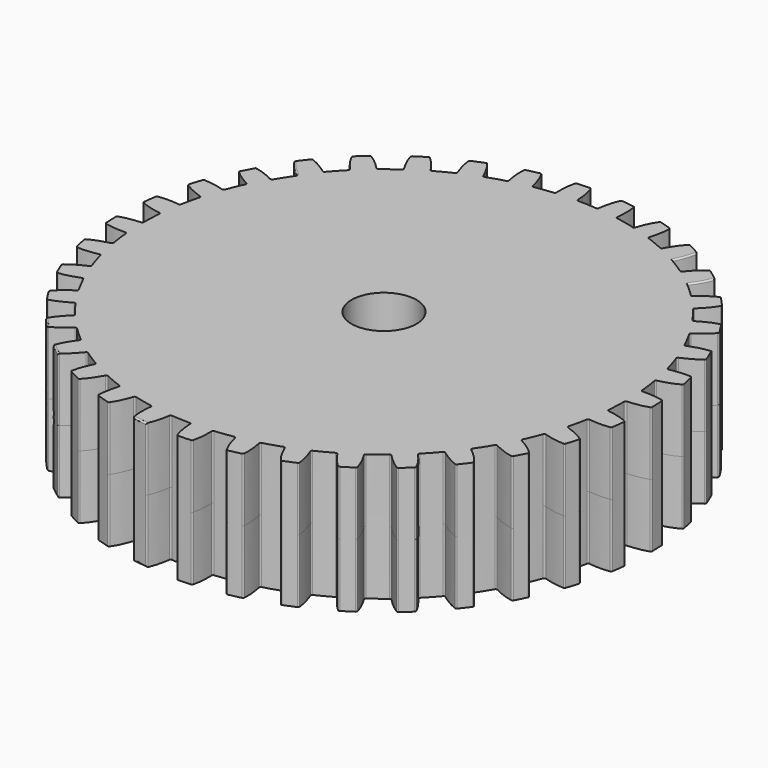
from build123d import *

# Parameters (mm, degrees)
F0_R     = 6.4021431983
F1_DEPTH = 12.5
F2_R     = 0.3


# Not quite as in the source:
# - the dataset's text gives a spline's control points without its knots; the knots are read off the source's solid


with BuildPart() as f1:
    # F0 (on Top) → F1 (new body, symmetric)
    with BuildSketch(Plane.XY):
        with BuildLine():
            ThreePointArc((47.3191638468, -4.1408613644), (47.4547694269, -2.0724040722), (47.5, 0))
            ThreePointArc((47.5, 0), (47.4999999975, 0.0004836327), (47.4999999902, 0.0009672655))
            ThreePointArc((47.4999999902, 0.0009672655), (47.4547905251, 2.0719208999), (47.3193324523, 4.1389341949))
            ThreePointArc((47.3193324523, 4.1389341949), (47.0936309153, 6.1999941305), (46.7782002945, 8.249241008))
            ThreePointArc((46.7782002945, 8.249241008), (46.3740603382, 10.2808816621), (45.8817270859, 12.2929703331))
            ThreePointArc((45.8817270859, 12.2929703331), (45.3015551605, 14.2835254765), (44.6350686538, 16.2468657368))
            ThreePointArc((44.6350686538, 16.2468657368), (43.8842777943, 18.1774630373), (43.0500286594, 20.0734907883))
            ThreePointArc((43.0500286594, 20.0734907883), (42.133014576, 21.9330591287), (41.1357230385, 23.7508376716))
            ThreePointArc((41.1357230385, 23.7508376716), (40.0610936761, 25.5217313965), (38.9102768963, 27.2440883835))
            ThreePointArc((38.9102768963, 27.2440883835), (37.6842836638, 28.9161678779), (36.3864892943, 30.5331524221))
            ThreePointArc((36.3864892943, 30.5331524221), (35.0206734985, 32.0905348617), (33.5882560594, 33.5868881394))
            ThreePointArc((33.5882560594, 33.5868881394), (32.0905348617, 35.0206734985), (30.5316704854, 36.3877327869))
            ThreePointArc((30.5316704854, 36.3877327869), (28.9161678779, 37.6842836638), (27.2456730585, 38.909167295))
            ThreePointArc((27.2456730585, 38.909167295), (25.5217313965, 40.0610936761), (23.7491623186, 41.136690304))
            ThreePointArc((23.7491623186, 41.136690304), (21.9330591287, 42.133014576), (20.0752440688, 43.0492110913))
            ThreePointArc((20.0752440688, 43.0492110913), (18.1774630373, 43.8842777943), (16.2450478724, 44.6357303024))
            ThreePointArc((16.2450478724, 44.6357303024), (14.2835254765, 45.3015551605), (12.2948389465, 45.8812263925))
            ThreePointArc((12.2948389465, 45.8812263925), (10.2808816621, 46.3740603382), (8.2473358669, 46.7785362223))
            ThreePointArc((8.2473358669, 46.7785362223), (6.1999941305, 47.0936309153), (4.1408613644, 47.3191638468))
            ThreePointArc((4.1408613644, 47.3191638468), (2.211991256, 47.4484677801), (0.2794571986, 47.4991779263))
            ThreePointArc((0.2794571986, 47.4991779263), (0.1392455732, 47.4997959014), (-0.0009672655, 47.4999999902))
            ThreePointArc((-0.0009672655, 47.4999999902), (-0.1402128345, 47.499793056), (-0.2794571986, 47.4991779263))
            ThreePointArc((-0.2794571986, 47.4991779263), (-2.2110250395, 47.4485128142), (-4.1389341949, 47.3193324523))
            ThreePointArc((-4.1389341949, 47.3193324523), (-6.1999941305, 47.0936309153), (-8.249241008, 46.7782002945))
            ThreePointArc((-8.249241008, 46.7782002945), (-10.2808816621, 46.3740603382), (-12.2929703331, 45.8817270859))
            ThreePointArc((-12.2929703331, 45.8817270859), (-14.2835254765, 45.3015551605), (-16.2468657368, 44.6350686538))
            ThreePointArc((-16.2468657368, 44.6350686538), (-18.1774630373, 43.8842777943), (-20.0734907883, 43.0500286594))
            ThreePointArc((-20.0734907883, 43.0500286594), (-21.9330591287, 42.133014576), (-23.7508376716, 41.1357230385))
            ThreePointArc((-23.7508376716, 41.1357230385), (-25.5217313965, 40.0610936761), (-27.2440883835, 38.9102768963))
            ThreePointArc((-27.2440883835, 38.9102768963), (-28.9161678779, 37.6842836638), (-30.5331524221, 36.3864892943))
            ThreePointArc((-30.5331524221, 36.3864892943), (-32.0905348617, 35.0206734985), (-33.5868881394, 33.5882560594))
            ThreePointArc((-33.5868881394, 33.5882560594), (-35.0206734985, 32.0905348617), (-36.3877327869, 30.5316704854))
            ThreePointArc((-36.3877327869, 30.5316704854), (-37.6842836638, 28.9161678779), (-38.909167295, 27.2456730585))
            ThreePointArc((-38.909167295, 27.2456730585), (-40.0610936761, 25.5217313965), (-41.136690304, 23.7491623186))
            ThreePointArc((-41.136690304, 23.7491623186), (-42.133014576, 21.9330591287), (-43.0492110913, 20.0752440688))
            ThreePointArc((-43.0492110913, 20.0752440688), (-43.8842777943, 18.1774630373), (-44.6357303024, 16.2450478724))
            ThreePointArc((-44.6357303024, 16.2450478724), (-45.3015551605, 14.2835254765), (-45.8812263925, 12.2948389465))
            ThreePointArc((-45.8812263925, 12.2948389465), (-46.3740603382, 10.2808816621), (-46.7785362223, 8.2473358669))
            ThreePointArc((-46.7785362223, 8.2473358669), (-47.0936309153, 6.1999941305), (-47.3191638468, 4.1408613644))
            ThreePointArc((-47.3191638468, 4.1408613644), (-47.4547905251, 2.0719208999), (-47.4999999902, -0.0009672655))
            ThreePointArc((-47.4999999902, -0.0009672655), (-47.4547905251, -2.0719208999), (-47.3193324523, -4.1389341949))
            ThreePointArc((-47.3193324523, -4.1389341949), (-47.0936309153, -6.1999941305), (-46.7782002945, -8.249241008))
            ThreePointArc((-46.7782002945, -8.249241008), (-46.3740603382, -10.2808816621), (-45.8817270859, -12.2929703331))
            ThreePointArc((-45.8817270859, -12.2929703331), (-45.3015551605, -14.2835254765), (-44.6350686538, -16.2468657368))
            ThreePointArc((-44.6350686538, -16.2468657368), (-43.8842777943, -18.1774630373), (-43.0500286594, -20.0734907883))
            ThreePointArc((-43.0500286594, -20.0734907883), (-42.133014576, -21.9330591287), (-41.1357230385, -23.7508376716))
            ThreePointArc((-41.1357230385, -23.7508376716), (-40.0610936761, -25.5217313965), (-38.9102768963, -27.2440883835))
            ThreePointArc((-38.9102768963, -27.2440883835), (-37.6842836638, -28.9161678779), (-36.3864892943, -30.5331524221))
            ThreePointArc((-36.3864892943, -30.5331524221), (-35.0206734985, -32.0905348617), (-33.5882560594, -33.5868881394))
            ThreePointArc((-33.5882560594, -33.5868881394), (-32.0905348617, -35.0206734985), (-30.5316704854, -36.3877327869))
            ThreePointArc((-30.5316704854, -36.3877327869), (-28.9161678779, -37.6842836638), (-27.2456730585, -38.909167295))
            ThreePointArc((-27.2456730585, -38.909167295), (-25.5217313965, -40.0610936761), (-23.7491623186, -41.136690304))
            ThreePointArc((-23.7491623186, -41.136690304), (-21.9330591287, -42.133014576), (-20.0752440688, -43.0492110913))
            ThreePointArc((-20.0752440688, -43.0492110913), (-18.1774630373, -43.8842777943), (-16.2450478724, -44.6357303024))
            ThreePointArc((-16.2450478724, -44.6357303024), (-14.2835254765, -45.3015551605), (-12.2948389465, -45.8812263925))
            ThreePointArc((-12.2948389465, -45.8812263925), (-10.2808816621, -46.3740603382), (-8.2473358669, -46.7785362223))
            ThreePointArc((-8.2473358669, -46.7785362223), (-6.1999941305, -47.0936309153), (-4.1408613644, -47.3191638468))
            ThreePointArc((-4.1408613644, -47.3191638468), (-2.0719208999, -47.4547905251), (0.0009672655, -47.4999999902))
            ThreePointArc((0.0009672655, -47.4999999902), (2.0719208999, -47.4547905251), (4.1389341949, -47.3193324523))
            ThreePointArc((4.1389341949, -47.3193324523), (6.1999941305, -47.0936309153), (8.249241008, -46.7782002945))
            ThreePointArc((8.249241008, -46.7782002945), (10.2808816621, -46.3740603382), (12.2929703331, -45.8817270859))
            ThreePointArc((12.2929703331, -45.8817270859), (14.2835254765, -45.3015551605), (16.2468657368, -44.6350686538))
            ThreePointArc((16.2468657368, -44.6350686538), (18.1774630373, -43.8842777943), (20.0734907883, -43.0500286594))
            ThreePointArc((20.0734907883, -43.0500286594), (21.9330591287, -42.133014576), (23.7508376716, -41.1357230385))
            ThreePointArc((23.7508376716, -41.1357230385), (25.5217313965, -40.0610936761), (27.2440883835, -38.9102768963))
            ThreePointArc((27.2440883835, -38.9102768963), (28.9161678779, -37.6842836638), (30.5331524221, -36.3864892943))
            ThreePointArc((30.5331524221, -36.3864892943), (32.0905348617, -35.0206734985), (33.5868881394, -33.5882560594))
            ThreePointArc((33.5868881394, -33.5882560594), (35.0206734985, -32.0905348617), (36.3877327869, -30.5316704854))
            ThreePointArc((36.3877327869, -30.5316704854), (37.6842836638, -28.9161678779), (38.909167295, -27.2456730585))
            ThreePointArc((38.909167295, -27.2456730585), (40.0610936761, -25.5217313965), (41.136690304, -23.7491623186))
            ThreePointArc((41.136690304, -23.7491623186), (42.133014576, -21.9330591287), (43.0492110913, -20.0752440688))
            ThreePointArc((43.0492110913, -20.0752440688), (43.8842777943, -18.1774630373), (44.6357303024, -16.2450478724))
            ThreePointArc((44.6357303024, -16.2450478724), (45.3015551605, -14.2835254765), (45.8812263925, -12.2948389465))
            ThreePointArc((45.8812263925, -12.2948389465), (46.3740603382, -10.2808816621), (46.7785362223, -8.2473358669))
            ThreePointArc((46.7785362223, -8.2473358669), (47.0936309153, -6.1999941305), (47.3191638468, -4.1408613644))
        make_face()
        Circle(F0_R, mode=Mode.SUBTRACT)
        with BuildLine():
            ThreePointArc((-43.0492110913, 20.0752440688), (-42.133014576, 21.9330591287), (-41.136690304, 23.7491623186))
            add(Edge.make_bspline(
                [(-45.4369608695, 25.2879929401), (-44.8516797618, 25.1784985185), (-43.3336628589, 24.8141226526), (-41.9586973612, 24.1177232288), (-41.136690304, 23.7491623186)],
                knots=[0.0012573797, 0.0012573797, 0.0012573797, 0.0012573797, 0.4755379839, 1, 1, 1, 1], degree=3))
            ThreePointArc((-45.4369608695, 25.2879929401), (-46.1245633253, 24.0109278882), (-46.7762812071, 22.7151825095))
            add(Edge.make_bspline(
                [(-46.7762812071, 22.7151825095), (-46.3508851757, 22.2985517138), (-45.1817072148, 21.2640624752), (-43.8226023929, 20.5371949767), (-43.0492110913, 20.0752440688)],
                knots=[0.0012573797, 0.0012573797, 0.0012573797, 0.0012573797, 0.4755379839, 1, 1, 1, 1], degree=3))
        make_face()
        with BuildLine():
            ThreePointArc((-45.8812263925, 12.2948389465), (-45.3015551605, 14.2835254765), (-44.6357303024, 16.2450478724))
            add(Edge.make_bspline(
                [(-49.1378852285, 17.0137660519), (-48.5424823492, 17.0075680943), (-46.9842543289, 16.9123287854), (-45.5092491558, 16.4652694867), (-44.6357303024, 16.2450478724)],
                knots=[0.0012573797, 0.0012573797, 0.0012573797, 0.0012573797, 0.4755379839, 1, 1, 1, 1], degree=3))
            ThreePointArc((-49.1378852285, 17.0137660519), (-49.5932814389, 15.6367015742), (-50.0100944379, 14.2474718568))
            add(Edge.make_bspline(
                [(-50.0100944379, 14.2474718568), (-49.5188139498, 13.9110398647), (-48.187761258, 13.0952924644), (-46.7230850757, 12.615473792), (-45.8812263925, 12.2948389465)],
                knots=[0.0012573797, 0.0012573797, 0.0012573797, 0.0012573797, 0.4755379839, 1, 1, 1, 1], degree=3))
        make_face()
        with BuildLine():
            ThreePointArc((-47.3191638468, 4.1408613644), (-47.0936309153, 6.1999941305), (-46.7785362223, 8.2473358669))
            add(Edge.make_bspline(
                [(-51.3457798098, 8.2225844915), (-50.7583461741, 8.3198713198), (-49.2072530063, 8.4966623661), (-47.6770254435, 8.312526863), (-46.7785362223, 8.2473358669)],
                knots=[0.0012573797, 0.0012573797, 0.0012573797, 0.0012573797, 0.4755379839, 1, 1, 1, 1], degree=3))
            ThreePointArc((-51.3457798098, 8.2225844915), (-51.5551327914, 6.7873619954), (-51.7243762556, 5.3468589813))
            add(Edge.make_bspline(
                [(-51.7243762556, 5.3468589813), (-51.1821386196, 5.1008481086), (-49.7296545597, 4.5286286186), (-48.2039104616, 4.3104378199), (-47.3191638468, 4.1408613644)],
                knots=[0.0012573797, 0.0012573797, 0.0012573797, 0.0012573797, 0.4755379839, 1, 1, 1, 1], degree=3))
        make_face()
        with BuildLine():
            add(Edge.make_bspline(
                [(-51.8670390746, -3.7162154987), (-51.290319907, -3.8643303361), (-49.7605374719, -4.1756353162), (-48.2200844205, -4.1255686242), (-47.3193324523, -4.1389341949)],
                knots=[0.0012573797, 0.0012573797, 0.0012573797, 0.0012573797, 0.4755379839, 1, 1, 1, 1], degree=3))
            ThreePointArc((-47.3193324523, -4.1389341949), (-47.4547905251, -2.0719208999), (-47.4999999902, -0.0009672655))
            add(Edge.make_bspline(
                [(-51.9935588538, -0.8184361379), (-51.4319433354, -0.6206205347), (-49.9351142012, -0.1771708397), (-48.3961594389, -0.092787683), (-47.4999999902, -0.0009672655)],
                knots=[0.0012573797, 0.0012573797, 0.0012573797, 0.0012573797, 0.4755379839, 1, 1, 1, 1], degree=3))
            ThreePointArc((-51.9935588538, -0.8184361379), (-51.9505075223, -2.268208143), (-51.8670390746, -3.7162154987))
        make_face()
        with BuildLine():
            add(Edge.make_bspline(
                [(-50.4337481573, -12.6663746513), (-49.8400707781, -12.712093059), (-48.2794716332, -12.7530246849), (-46.7711155148, -12.4362217532), (-45.8817270859, -12.2929703331)],
                knots=[0.0012573797, 0.0012573797, 0.0012573797, 0.0012573797, 0.4755379839, 1, 1, 1, 1], degree=3))
            ThreePointArc((-45.8817270859, -12.2929703331), (-46.3740603382, -10.2808816621), (-46.7782002945, -8.249241008))
            add(Edge.make_bspline(
                [(-51.0615399221, -9.8345889993), (-50.5428069243, -9.5422551483), (-49.1457222194, -8.8456207992), (-47.6448006194, -8.4952829223), (-46.7782002945, -8.249241008)],
                knots=[0.0012573797, 0.0012573797, 0.0012573797, 0.0012573797, 0.4755379839, 1, 1, 1, 1], degree=3))
            ThreePointArc((-51.0615399221, -9.8345889993), (-50.7673923702, -11.2548599248), (-50.4337481573, -12.6663746513))
        make_face()
        with BuildLine():
            add(Edge.make_bspline(
                [(-47.4680533229, -21.2316724196), (-46.8754563189, -21.173605267), (-45.3314584794, -20.9429198518), (-43.9010299315, -20.3690065773), (-43.0500286594, -20.0734907883)],
                knots=[0.0012573797, 0.0012573797, 0.0012573797, 0.0012573797, 0.4755379839, 1, 1, 1, 1], degree=3))
            ThreePointArc((-43.0500286594, -20.0734907883), (-43.8842777943, -18.1774630373), (-44.6350686538, -16.2468657368))
            add(Edge.make_bspline(
                [(-48.5780419382, -18.5519228506), (-48.1179529007, -18.1739531679), (-46.8630623369, -17.2453010468), (-45.4457786425, -16.6396532887), (-44.6350686538, -16.2468657368)],
                knots=[0.0012573797, 0.0012573797, 0.0012573797, 0.0012573797, 0.4755379839, 1, 1, 1, 1], degree=3))
            ThreePointArc((-48.5780419382, -18.5519228506), (-48.0417356906, -19.899538483), (-47.4680533229, -21.2316724196))
        make_face()
        with BuildLine():
            add(Edge.make_bspline(
                [(-43.0600657083, -29.1518565651), (-42.4865548396, -28.9917681932), (-41.0060718986, -28.4964749967), (-39.6970337687, -27.6828894438), (-38.9102768963, -27.2440883835)],
                knots=[0.0012573797, 0.0012573797, 0.0012573797, 0.0012573797, 0.4755379839, 1, 1, 1, 1], degree=3))
            ThreePointArc((-38.9102768963, -27.2440883835), (-40.0610936761, -25.5217313965), (-41.1357230385, -23.7508376716))
            add(Edge.make_bspline(
                [(-44.6185247317, -26.7055659137), (-44.2310592271, -26.2534448169), (-43.1564920192, -25.1209915486), (-41.8659096782, -24.2784362101), (-41.1357230385, -23.7508376716)],
                knots=[0.0012573797, 0.0012573797, 0.0012573797, 0.0012573797, 0.4755379839, 1, 1, 1, 1], degree=3))
            ThreePointArc((-44.6185247317, -26.7055659137), (-43.8563551823, -27.939579634), (-43.0600657083, -29.1518565651))
        make_face()
        with BuildLine():
            add(Edge.make_bspline(
                [(-37.3437197866, -36.1862763005), (-36.8067208907, -35.9290309134), (-35.4347365732, -35.1841791688), (-34.2868633225, -34.1556417228), (-33.5882560594, -33.5868881394)],
                knots=[0.0012573797, 0.0012573797, 0.0012573797, 0.0012573797, 0.4755379839, 1, 1, 1, 1], degree=3))
            ThreePointArc((-33.5882560594, -33.5868881394), (-35.0206734985, -32.0905348617), (-36.3864892943, -30.5331524221))
            add(Edge.make_bspline(
                [(-39.3032962292, -34.0477738702), (-39.0002272009, -33.53523883), (-38.1386335297, -32.233393434), (-37.0139662335, -31.1795311327), (-36.3864892943, -30.5331524221)],
                knots=[0.0012573797, 0.0012573797, 0.0012573797, 0.0012573797, 0.4755379839, 1, 1, 1, 1], degree=3))
            ThreePointArc((-39.3032962292, -34.0477738702), (-38.3384215141, -35.130690796), (-37.3437197866, -36.1862763005))
        make_face()
        with BuildLine():
            add(Edge.make_bspline(
                [(-30.4927038361, -42.1211943416), (-30.0085333527, -41.7746082103), (-28.7867347078, -40.8028298608), (-27.8349038843, -39.5905921116), (-27.2456730585, -38.909167295)],
                knots=[0.0012573797, 0.0012573797, 0.0012573797, 0.0012573797, 0.4755379839, 1, 1, 1, 1], degree=3))
            ThreePointArc((-27.2456730585, -38.909167295), (-28.9161678779, -37.6842836638), (-30.5316704854, -36.3877327869))
            add(Edge.make_bspline(
                [(-32.7938569593, -40.3554574467), (-32.5843930062, -39.798081581), (-31.9619519595, -38.3663999709), (-31.0373721548, -37.1332517795), (-30.5316704854, -36.3877327869)],
                knots=[0.0012573797, 0.0012573797, 0.0012573797, 0.0012573797, 0.4755379839, 1, 1, 1, 1], degree=3))
            ThreePointArc((-32.7938569593, -40.3554574467), (-31.6555943085, -41.2543736951), (-30.4927038361, -42.1211943416))
        make_face()
        with BuildLine():
            add(Edge.make_bspline(
                [(-22.7151825095, -46.7762812071), (-22.2985517138, -46.3508851757), (-21.2640624752, -45.1817072148), (-20.5371949767, -43.8226023929), (-20.0752440688, -43.0492110913)],
                knots=[0.0012573797, 0.0012573797, 0.0012573797, 0.0012573797, 0.4755379839, 1, 1, 1, 1], degree=3))
            ThreePointArc((-20.0752440688, -43.0492110913), (-21.9330591287, -42.133014576), (-23.7491623186, -41.136690304))
            add(Edge.make_bspline(
                [(-25.2879929401, -45.4369608695), (-25.1784985185, -44.8516797618), (-24.8141226526, -43.3336628589), (-24.1177232288, -41.9586973612), (-23.7491623186, -41.136690304)],
                knots=[0.0012573797, 0.0012573797, 0.0012573797, 0.0012573797, 0.4755379839, 1, 1, 1, 1], degree=3))
            ThreePointArc((-25.2879929401, -45.4369608695), (-24.0109278882, -46.1245633253), (-22.7151825095, -46.7762812071))
        make_face()
        with BuildLine():
            add(Edge.make_bspline(
                [(-14.2474718568, -50.0100944379), (-13.9110398647, -49.5188139498), (-13.0952924644, -48.187761258), (-12.615473792, -46.7230850757), (-12.2948389465, -45.8812263925)],
                knots=[0.0012573797, 0.0012573797, 0.0012573797, 0.0012573797, 0.4755379839, 1, 1, 1, 1], degree=3))
            ThreePointArc((-12.2948389465, -45.8812263925), (-14.2835254765, -45.3015551605), (-16.2450478724, -44.6357303024))
            add(Edge.make_bspline(
                [(-17.0137660519, -49.1378852285), (-17.0075680943, -48.5424823492), (-16.9123287854, -46.9842543289), (-16.4652694867, -45.5092491558), (-16.2450478724, -44.6357303024)],
                knots=[0.0012573797, 0.0012573797, 0.0012573797, 0.0012573797, 0.4755379839, 1, 1, 1, 1], degree=3))
            ThreePointArc((-17.0137660519, -49.1378852285), (-15.6367015742, -49.5932814389), (-14.2474718568, -50.0100944379))
        make_face()
        with BuildLine():
            add(Edge.make_bspline(
                [(-5.3468589813, -51.7243762556), (-5.1008481086, -51.1821386196), (-4.5286286186, -49.7296545597), (-4.3104378199, -48.2039104616), (-4.1408613644, -47.3191638468)],
                knots=[0.0012573797, 0.0012573797, 0.0012573797, 0.0012573797, 0.4755379839, 1, 1, 1, 1], degree=3))
            ThreePointArc((-4.1408613644, -47.3191638468), (-6.1999941305, -47.0936309153), (-8.2473358669, -46.7785362223))
            add(Edge.make_bspline(
                [(-8.2225844915, -51.3457798098), (-8.3198713198, -50.7583461741), (-8.4966623661, -49.2072530063), (-8.312526863, -47.6770254435), (-8.2473358669, -46.7785362223)],
                knots=[0.0012573797, 0.0012573797, 0.0012573797, 0.0012573797, 0.4755379839, 1, 1, 1, 1], degree=3))
            ThreePointArc((-8.2225844915, -51.3457798098), (-6.7873619954, -51.5551327914), (-5.3468589813, -51.7243762556))
        make_face()
        with BuildLine():
            add(Edge.make_bspline(
                [(3.7162154987, -51.8670390746), (3.8643303361, -51.290319907), (4.1756353162, -49.7605374719), (4.1255686242, -48.2200844205), (4.1389341949, -47.3193324523)],
                knots=[0.0012573797, 0.0012573797, 0.0012573797, 0.0012573797, 0.4755379839, 1, 1, 1, 1], degree=3))
            ThreePointArc((4.1389341949, -47.3193324523), (2.0719208999, -47.4547905251), (0.0009672655, -47.4999999902))
            add(Edge.make_bspline(
                [(0.8184361379, -51.9935588538), (0.6206205347, -51.4319433354), (0.1771708397, -49.9351142012), (0.092787683, -48.3961594389), (0.0009672655, -47.4999999902)],
                knots=[0.0012573797, 0.0012573797, 0.0012573797, 0.0012573797, 0.4755379839, 1, 1, 1, 1], degree=3))
            ThreePointArc((0.8184361379, -51.9935588538), (2.268208143, -51.9505075223), (3.7162154987, -51.8670390746))
        make_face()
        with BuildLine():
            add(Edge.make_bspline(
                [(12.6663746513, -50.4337481573), (12.712093059, -49.8400707781), (12.7530246849, -48.2794716332), (12.4362217532, -46.7711155148), (12.2929703331, -45.8817270859)],
                knots=[0.0012573797, 0.0012573797, 0.0012573797, 0.0012573797, 0.4755379839, 1, 1, 1, 1], degree=3))
            ThreePointArc((12.2929703331, -45.8817270859), (10.2808816621, -46.3740603382), (8.249241008, -46.7782002945))
            add(Edge.make_bspline(
                [(9.8345889993, -51.0615399221), (9.5422551483, -50.5428069243), (8.8456207992, -49.1457222194), (8.4952829223, -47.6448006194), (8.249241008, -46.7782002945)],
                knots=[0.0012573797, 0.0012573797, 0.0012573797, 0.0012573797, 0.4755379839, 1, 1, 1, 1], degree=3))
            ThreePointArc((9.8345889993, -51.0615399221), (11.2548599248, -50.7673923702), (12.6663746513, -50.4337481573))
        make_face()
        with BuildLine():
            add(Edge.make_bspline(
                [(21.2316724196, -47.4680533229), (21.173605267, -46.8754563189), (20.9429198518, -45.3314584794), (20.3690065773, -43.9010299315), (20.0734907883, -43.0500286594)],
                knots=[0.0012573797, 0.0012573797, 0.0012573797, 0.0012573797, 0.4755379839, 1, 1, 1, 1], degree=3))
            ThreePointArc((20.0734907883, -43.0500286594), (18.1774630373, -43.8842777943), (16.2468657368, -44.6350686538))
            add(Edge.make_bspline(
                [(18.5519228506, -48.5780419382), (18.1739531679, -48.1179529007), (17.2453010468, -46.8630623369), (16.6396532887, -45.4457786425), (16.2468657368, -44.6350686538)],
                knots=[0.0012573797, 0.0012573797, 0.0012573797, 0.0012573797, 0.4755379839, 1, 1, 1, 1], degree=3))
            ThreePointArc((18.5519228506, -48.5780419382), (19.899538483, -48.0417356906), (21.2316724196, -47.4680533229))
        make_face()
        with BuildLine():
            add(Edge.make_bspline(
                [(29.1518565651, -43.0600657083), (28.9917681932, -42.4865548396), (28.4964749967, -41.0060718986), (27.6828894438, -39.6970337687), (27.2440883835, -38.9102768963)],
                knots=[0.0012573797, 0.0012573797, 0.0012573797, 0.0012573797, 0.4755379839, 1, 1, 1, 1], degree=3))
            ThreePointArc((27.2440883835, -38.9102768963), (25.5217313965, -40.0610936761), (23.7508376716, -41.1357230385))
            add(Edge.make_bspline(
                [(26.7055659137, -44.6185247317), (26.2534448169, -44.2310592271), (25.1209915486, -43.1564920192), (24.2784362101, -41.8659096782), (23.7508376716, -41.1357230385)],
                knots=[0.0012573797, 0.0012573797, 0.0012573797, 0.0012573797, 0.4755379839, 1, 1, 1, 1], degree=3))
            ThreePointArc((26.7055659137, -44.6185247317), (27.939579634, -43.8563551823), (29.1518565651, -43.0600657083))
        make_face()
        with BuildLine():
            add(Edge.make_bspline(
                [(36.1862763005, -37.3437197866), (35.9290309134, -36.8067208907), (35.1841791688, -35.4347365732), (34.1556417228, -34.2868633225), (33.5868881394, -33.5882560594)],
                knots=[0.0012573797, 0.0012573797, 0.0012573797, 0.0012573797, 0.4755379839, 1, 1, 1, 1], degree=3))
            ThreePointArc((33.5868881394, -33.5882560594), (32.0905348617, -35.0206734985), (30.5331524221, -36.3864892943))
            add(Edge.make_bspline(
                [(34.0477738702, -39.3032962292), (33.53523883, -39.0002272009), (32.233393434, -38.1386335297), (31.1795311327, -37.0139662335), (30.5331524221, -36.3864892943)],
                knots=[0.0012573797, 0.0012573797, 0.0012573797, 0.0012573797, 0.4755379839, 1, 1, 1, 1], degree=3))
            ThreePointArc((34.0477738702, -39.3032962292), (35.130690796, -38.3384215141), (36.1862763005, -37.3437197866))
        make_face()
        with BuildLine():
            add(Edge.make_bspline(
                [(42.1211943416, -30.4927038361), (41.7746082103, -30.0085333527), (40.8028298608, -28.7867347078), (39.5905921116, -27.8349038843), (38.909167295, -27.2456730585)],
                knots=[0.0012573797, 0.0012573797, 0.0012573797, 0.0012573797, 0.4755379839, 1, 1, 1, 1], degree=3))
            ThreePointArc((38.909167295, -27.2456730585), (37.6842836638, -28.9161678779), (36.3877327869, -30.5316704854))
            add(Edge.make_bspline(
                [(40.3554574467, -32.7938569593), (39.798081581, -32.5843930062), (38.3663999709, -31.9619519595), (37.1332517795, -31.0373721548), (36.3877327869, -30.5316704854)],
                knots=[0.0012573797, 0.0012573797, 0.0012573797, 0.0012573797, 0.4755379839, 1, 1, 1, 1], degree=3))
            ThreePointArc((40.3554574467, -32.7938569593), (41.2543736951, -31.6555943085), (42.1211943416, -30.4927038361))
        make_face()
        with BuildLine():
            ThreePointArc((-27.2440883835, 38.9102768963), (-25.5217313965, 40.0610936761), (-23.7508376716, 41.1357230385))
            add(Edge.make_bspline(
                [(-26.7055659137, 44.6185247317), (-26.2534448169, 44.2310592271), (-25.1209915486, 43.1564920192), (-24.2784362101, 41.8659096782), (-23.7508376716, 41.1357230385)],
                knots=[0.0012573797, 0.0012573797, 0.0012573797, 0.0012573797, 0.4755379839, 1, 1, 1, 1], degree=3))
            ThreePointArc((-26.7055659137, 44.6185247317), (-27.939579634, 43.8563551823), (-29.1518565651, 43.0600657083))
            add(Edge.make_bspline(
                [(-29.1518565651, 43.0600657083), (-28.9917681932, 42.4865548396), (-28.4964749967, 41.0060718986), (-27.6828894438, 39.6970337687), (-27.2440883835, 38.9102768963)],
                knots=[0.0012573797, 0.0012573797, 0.0012573797, 0.0012573797, 0.4755379839, 1, 1, 1, 1], degree=3))
        make_face()
        with BuildLine():
            add(Edge.make_bspline(
                [(50.0100944379, -14.2474718568), (49.5188139498, -13.9110398647), (48.187761258, -13.0952924644), (46.7230850757, -12.615473792), (45.8812263925, -12.2948389465)],
                knots=[0.0012573797, 0.0012573797, 0.0012573797, 0.0012573797, 0.4755379839, 1, 1, 1, 1], degree=3))
            ThreePointArc((45.8812263925, -12.2948389465), (45.3015551605, -14.2835254765), (44.6357303024, -16.2450478724))
            add(Edge.make_bspline(
                [(49.1378852285, -17.0137660519), (48.5424823492, -17.0075680943), (46.9842543289, -16.9123287854), (45.5092491558, -16.4652694867), (44.6357303024, -16.2450478724)],
                knots=[0.0012573797, 0.0012573797, 0.0012573797, 0.0012573797, 0.4755379839, 1, 1, 1, 1], degree=3))
            ThreePointArc((49.1378852285, -17.0137660519), (49.5932814389, -15.6367015742), (50.0100944379, -14.2474718568))
        make_face()
        with BuildLine():
            ThreePointArc((12.2948389465, 45.8812263925), (14.2835254765, 45.3015551605), (16.2450478724, 44.6357303024))
            add(Edge.make_bspline(
                [(17.0137660519, 49.1378852285), (17.0075680943, 48.5424823492), (16.9123287854, 46.9842543289), (16.4652694867, 45.5092491558), (16.2450478724, 44.6357303024)],
                knots=[0.0012573797, 0.0012573797, 0.0012573797, 0.0012573797, 0.4755379839, 1, 1, 1, 1], degree=3))
            ThreePointArc((17.0137660519, 49.1378852285), (15.6367015742, 49.5932814389), (14.2474718568, 50.0100944379))
            add(Edge.make_bspline(
                [(14.2474718568, 50.0100944379), (13.9110398647, 49.5188139498), (13.0952924644, 48.187761258), (12.615473792, 46.7230850757), (12.2948389465, 45.8812263925)],
                knots=[0.0012573797, 0.0012573797, 0.0012573797, 0.0012573797, 0.4755379839, 1, 1, 1, 1], degree=3))
        make_face()
        with BuildLine():
            ThreePointArc((-4.1389341949, 47.3193324523), (-2.2110250395, 47.4485128142), (-0.2794571986, 47.4991779263))
            add(Edge.make_bspline(
                [(-0.1401693003, 48.9738556219), (-0.1894884148, 48.5017472335), (-0.2266014064, 48.0150459528), (-0.2794571986, 47.4991779263)],
                knots=[0.6980970455, 0.6980970455, 0.6980970455, 0.6980970455, 1, 1, 1, 1], degree=3))
            add(Edge.make_bspline(
                [(-0.8184361379, 51.9935588538), (-0.6206205347, 51.4319433354), (-0.3111403588, 50.387317645), (-0.17654491, 49.3221745068), (-0.1401693003, 48.9738556219)],
                knots=[0.0012573797, 0.0012573797, 0.0012573797, 0.0012573797, 0.4755379839, 0.698272273, 0.698272273, 0.698272273, 0.698272273], degree=3))
            ThreePointArc((-0.8184361379, 51.9935588538), (-2.268208143, 51.9505075223), (-3.7162154987, 51.8670390746))
            add(Edge.make_bspline(
                [(-3.7162154987, 51.8670390746), (-3.8643303361, 51.290319907), (-4.1756353162, 49.7605374719), (-4.1255686242, 48.2200844205), (-4.1389341949, 47.3193324523)],
                knots=[0.0012573797, 0.0012573797, 0.0012573797, 0.0012573797, 0.4755379839, 1, 1, 1, 1], degree=3))
        make_face()
        with BuildLine():
            ThreePointArc((-12.2929703331, 45.8817270859), (-10.2808816621, 46.3740603382), (-8.249241008, 46.7782002945))
            add(Edge.make_bspline(
                [(-9.8345889993, 51.0615399221), (-9.5422551483, 50.5428069243), (-8.8456207992, 49.1457222194), (-8.4952829223, 47.6448006194), (-8.249241008, 46.7782002945)],
                knots=[0.0012573797, 0.0012573797, 0.0012573797, 0.0012573797, 0.4755379839, 1, 1, 1, 1], degree=3))
            ThreePointArc((-9.8345889993, 51.0615399221), (-11.2548599248, 50.7673923702), (-12.6663746513, 50.4337481573))
            add(Edge.make_bspline(
                [(-12.6663746513, 50.4337481573), (-12.712093059, 49.8400707781), (-12.7530246849, 48.2794716332), (-12.4362217532, 46.7711155148), (-12.2929703331, 45.8817270859)],
                knots=[0.0012573797, 0.0012573797, 0.0012573797, 0.0012573797, 0.4755379839, 1, 1, 1, 1], degree=3))
        make_face()
        with BuildLine():
            ThreePointArc((-38.909167295, 27.2456730585), (-37.6842836638, 28.9161678779), (-36.3877327869, 30.5316704854))
            add(Edge.make_bspline(
                [(-40.3554574467, 32.7938569593), (-39.798081581, 32.5843930062), (-38.3663999709, 31.9619519595), (-37.1332517795, 31.0373721548), (-36.3877327869, 30.5316704854)],
                knots=[0.0012573797, 0.0012573797, 0.0012573797, 0.0012573797, 0.4755379839, 1, 1, 1, 1], degree=3))
            ThreePointArc((-40.3554574467, 32.7938569593), (-41.2543736951, 31.6555943085), (-42.1211943416, 30.4927038361))
            add(Edge.make_bspline(
                [(-42.1211943416, 30.4927038361), (-41.7746082103, 30.0085333527), (-40.8028298608, 28.7867347078), (-39.5905921116, 27.8349038843), (-38.909167295, 27.2456730585)],
                knots=[0.0012573797, 0.0012573797, 0.0012573797, 0.0012573797, 0.4755379839, 1, 1, 1, 1], degree=3))
        make_face()
        with BuildLine():
            ThreePointArc((-0.2794571986, 47.4991779263), (-0.1402128345, 47.499793056), (-0.0009672655, 47.4999999902))
            add(Edge.make_bspline(
                [(-0.1401693003, 48.9738556219), (-0.0908929625, 48.5020043151), (-0.0537923796, 48.0155686018), (-0.0009672655, 47.4999999902)],
                knots=[0.698272273, 0.698272273, 0.698272273, 0.698272273, 1, 1, 1, 1], degree=3))
            add(Edge.make_bspline(
                [(-0.1401693003, 48.9738556219), (-0.1894884148, 48.5017472335), (-0.2266014064, 48.0150459528), (-0.2794571986, 47.4991779263)],
                knots=[0.6980970455, 0.6980970455, 0.6980970455, 0.6980970455, 1, 1, 1, 1], degree=3))
        make_face()
        with BuildLine():
            add(Edge.make_bspline(
                [(46.7762812071, -22.7151825095), (46.3508851757, -22.2985517138), (45.1817072148, -21.2640624752), (43.8226023929, -20.5371949767), (43.0492110913, -20.0752440688)],
                knots=[0.0012573797, 0.0012573797, 0.0012573797, 0.0012573797, 0.4755379839, 1, 1, 1, 1], degree=3))
            ThreePointArc((43.0492110913, -20.0752440688), (42.133014576, -21.9330591287), (41.136690304, -23.7491623186))
            add(Edge.make_bspline(
                [(45.4369608695, -25.2879929401), (44.8516797618, -25.1784985185), (43.3336628589, -24.8141226526), (41.9586973612, -24.1177232288), (41.136690304, -23.7491623186)],
                knots=[0.0012573797, 0.0012573797, 0.0012573797, 0.0012573797, 0.4755379839, 1, 1, 1, 1], degree=3))
            ThreePointArc((45.4369608695, -25.2879929401), (46.1245633253, -24.0109278882), (46.7762812071, -22.7151825095))
        make_face()
        with BuildLine():
            add(Edge.make_bspline(
                [(51.7243762556, -5.3468589813), (51.1821386196, -5.1008481086), (49.7296545597, -4.5286286186), (48.2039104616, -4.3104378199), (47.3191638468, -4.1408613644)],
                knots=[0.0012573797, 0.0012573797, 0.0012573797, 0.0012573797, 0.4755379839, 1, 1, 1, 1], degree=3))
            ThreePointArc((47.3191638468, -4.1408613644), (47.0936309153, -6.1999941305), (46.7785362223, -8.2473358669))
            add(Edge.make_bspline(
                [(51.3457798098, -8.2225844915), (50.7583461741, -8.3198713198), (49.2072530063, -8.4966623661), (47.6770254435, -8.312526863), (46.7785362223, -8.2473358669)],
                knots=[0.0012573797, 0.0012573797, 0.0012573797, 0.0012573797, 0.4755379839, 1, 1, 1, 1], degree=3))
            ThreePointArc((51.3457798098, -8.2225844915), (51.5551327914, -6.7873619954), (51.7243762556, -5.3468589813))
        make_face()
        with BuildLine():
            ThreePointArc((47.3193324523, 4.1389341949), (47.4547905251, 2.0719208999), (47.4999999902, 0.0009672655))
            add(Edge.make_bspline(
                [(51.9935588538, 0.8184361379), (51.4319433354, 0.6206205347), (49.9351142012, 0.1771708397), (48.3961594389, 0.092787683), (47.4999999902, 0.0009672655)],
                knots=[0.0012573797, 0.0012573797, 0.0012573797, 0.0012573797, 0.4755379839, 1, 1, 1, 1], degree=3))
            ThreePointArc((51.9935588538, 0.8184361379), (51.9505075223, 2.268208143), (51.8670390746, 3.7162154987))
            add(Edge.make_bspline(
                [(51.8670390746, 3.7162154987), (51.290319907, 3.8643303361), (49.7605374719, 4.1756353162), (48.2200844205, 4.1255686242), (47.3193324523, 4.1389341949)],
                knots=[0.0012573797, 0.0012573797, 0.0012573797, 0.0012573797, 0.4755379839, 1, 1, 1, 1], degree=3))
        make_face()
        with BuildLine():
            ThreePointArc((45.8817270859, 12.2929703331), (46.3740603382, 10.2808816621), (46.7782002945, 8.249241008))
            add(Edge.make_bspline(
                [(51.0615399221, 9.8345889993), (50.5428069243, 9.5422551483), (49.1457222194, 8.8456207992), (47.6448006194, 8.4952829223), (46.7782002945, 8.249241008)],
                knots=[0.0012573797, 0.0012573797, 0.0012573797, 0.0012573797, 0.4755379839, 1, 1, 1, 1], degree=3))
            ThreePointArc((51.0615399221, 9.8345889993), (50.7673923702, 11.2548599248), (50.4337481573, 12.6663746513))
            add(Edge.make_bspline(
                [(50.4337481573, 12.6663746513), (49.8400707781, 12.712093059), (48.2794716332, 12.7530246849), (46.7711155148, 12.4362217532), (45.8817270859, 12.2929703331)],
                knots=[0.0012573797, 0.0012573797, 0.0012573797, 0.0012573797, 0.4755379839, 1, 1, 1, 1], degree=3))
        make_face()
        with BuildLine():
            ThreePointArc((43.0500286594, 20.0734907883), (43.8842777943, 18.1774630373), (44.6350686538, 16.2468657368))
            add(Edge.make_bspline(
                [(48.5780419382, 18.5519228506), (48.1179529007, 18.1739531679), (46.8630623369, 17.2453010468), (45.4457786425, 16.6396532887), (44.6350686538, 16.2468657368)],
                knots=[0.0012573797, 0.0012573797, 0.0012573797, 0.0012573797, 0.4755379839, 1, 1, 1, 1], degree=3))
            ThreePointArc((48.5780419382, 18.5519228506), (48.0417356906, 19.899538483), (47.4680533229, 21.2316724196))
            add(Edge.make_bspline(
                [(47.4680533229, 21.2316724196), (46.8754563189, 21.173605267), (45.3314584794, 20.9429198518), (43.9010299315, 20.3690065773), (43.0500286594, 20.0734907883)],
                knots=[0.0012573797, 0.0012573797, 0.0012573797, 0.0012573797, 0.4755379839, 1, 1, 1, 1], degree=3))
        make_face()
        with BuildLine():
            ThreePointArc((38.9102768963, 27.2440883835), (40.0610936761, 25.5217313965), (41.1357230385, 23.7508376716))
            add(Edge.make_bspline(
                [(44.6185247317, 26.7055659137), (44.2310592271, 26.2534448169), (43.1564920192, 25.1209915486), (41.8659096782, 24.2784362101), (41.1357230385, 23.7508376716)],
                knots=[0.0012573797, 0.0012573797, 0.0012573797, 0.0012573797, 0.4755379839, 1, 1, 1, 1], degree=3))
            ThreePointArc((44.6185247317, 26.7055659137), (43.8563551823, 27.939579634), (43.0600657083, 29.1518565651))
            add(Edge.make_bspline(
                [(43.0600657083, 29.1518565651), (42.4865548396, 28.9917681932), (41.0060718986, 28.4964749967), (39.6970337687, 27.6828894438), (38.9102768963, 27.2440883835)],
                knots=[0.0012573797, 0.0012573797, 0.0012573797, 0.0012573797, 0.4755379839, 1, 1, 1, 1], degree=3))
        make_face()
        with BuildLine():
            ThreePointArc((33.5882560594, 33.5868881394), (35.0206734985, 32.0905348617), (36.3864892943, 30.5331524221))
            add(Edge.make_bspline(
                [(39.3032962292, 34.0477738702), (39.0002272009, 33.53523883), (38.1386335297, 32.233393434), (37.0139662335, 31.1795311327), (36.3864892943, 30.5331524221)],
                knots=[0.0012573797, 0.0012573797, 0.0012573797, 0.0012573797, 0.4755379839, 1, 1, 1, 1], degree=3))
            ThreePointArc((39.3032962292, 34.0477738702), (38.3384215141, 35.130690796), (37.3437197866, 36.1862763005))
            add(Edge.make_bspline(
                [(37.3437197866, 36.1862763005), (36.8067208907, 35.9290309134), (35.4347365732, 35.1841791688), (34.2868633225, 34.1556417228), (33.5882560594, 33.5868881394)],
                knots=[0.0012573797, 0.0012573797, 0.0012573797, 0.0012573797, 0.4755379839, 1, 1, 1, 1], degree=3))
        make_face()
        with BuildLine():
            ThreePointArc((27.2456730585, 38.909167295), (28.9161678779, 37.6842836638), (30.5316704854, 36.3877327869))
            add(Edge.make_bspline(
                [(32.7938569593, 40.3554574467), (32.5843930062, 39.798081581), (31.9619519595, 38.3663999709), (31.0373721548, 37.1332517795), (30.5316704854, 36.3877327869)],
                knots=[0.0012573797, 0.0012573797, 0.0012573797, 0.0012573797, 0.4755379839, 1, 1, 1, 1], degree=3))
            ThreePointArc((32.7938569593, 40.3554574467), (31.6555943085, 41.2543736951), (30.4927038361, 42.1211943416))
            add(Edge.make_bspline(
                [(30.4927038361, 42.1211943416), (30.0085333527, 41.7746082103), (28.7867347078, 40.8028298608), (27.8349038843, 39.5905921116), (27.2456730585, 38.909167295)],
                knots=[0.0012573797, 0.0012573797, 0.0012573797, 0.0012573797, 0.4755379839, 1, 1, 1, 1], degree=3))
        make_face()
        with BuildLine():
            ThreePointArc((20.0752440688, 43.0492110913), (21.9330591287, 42.133014576), (23.7491623186, 41.136690304))
            add(Edge.make_bspline(
                [(25.2879929401, 45.4369608695), (25.1784985185, 44.8516797618), (24.8141226526, 43.3336628589), (24.1177232288, 41.9586973612), (23.7491623186, 41.136690304)],
                knots=[0.0012573797, 0.0012573797, 0.0012573797, 0.0012573797, 0.4755379839, 1, 1, 1, 1], degree=3))
            ThreePointArc((25.2879929401, 45.4369608695), (24.0109278882, 46.1245633253), (22.7151825095, 46.7762812071))
            add(Edge.make_bspline(
                [(22.7151825095, 46.7762812071), (22.2985517138, 46.3508851757), (21.2640624752, 45.1817072148), (20.5371949767, 43.8226023929), (20.0752440688, 43.0492110913)],
                knots=[0.0012573797, 0.0012573797, 0.0012573797, 0.0012573797, 0.4755379839, 1, 1, 1, 1], degree=3))
        make_face()
        with BuildLine():
            ThreePointArc((4.1408613644, 47.3191638468), (6.1999941305, 47.0936309153), (8.2473358669, 46.7785362223))
            add(Edge.make_bspline(
                [(8.2225844915, 51.3457798098), (8.3198713198, 50.7583461741), (8.4966623661, 49.2072530063), (8.312526863, 47.6770254435), (8.2473358669, 46.7785362223)],
                knots=[0.0012573797, 0.0012573797, 0.0012573797, 0.0012573797, 0.4755379839, 1, 1, 1, 1], degree=3))
            ThreePointArc((8.2225844915, 51.3457798098), (6.7873619954, 51.5551327914), (5.3468589813, 51.7243762556))
            add(Edge.make_bspline(
                [(5.3468589813, 51.7243762556), (5.1008481086, 51.1821386196), (4.5286286186, 49.7296545597), (4.3104378199, 48.2039104616), (4.1408613644, 47.3191638468)],
                knots=[0.0012573797, 0.0012573797, 0.0012573797, 0.0012573797, 0.4755379839, 1, 1, 1, 1], degree=3))
        make_face()
        with BuildLine():
            ThreePointArc((-20.0734907883, 43.0500286594), (-18.1774630373, 43.8842777943), (-16.2468657368, 44.6350686538))
            add(Edge.make_bspline(
                [(-18.5519228506, 48.5780419382), (-18.1739531679, 48.1179529007), (-17.2453010468, 46.8630623369), (-16.6396532887, 45.4457786425), (-16.2468657368, 44.6350686538)],
                knots=[0.0012573797, 0.0012573797, 0.0012573797, 0.0012573797, 0.4755379839, 1, 1, 1, 1], degree=3))
            ThreePointArc((-18.5519228506, 48.5780419382), (-19.899538483, 48.0417356906), (-21.2316724196, 47.4680533229))
            add(Edge.make_bspline(
                [(-21.2316724196, 47.4680533229), (-21.173605267, 46.8754563189), (-20.9429198518, 45.3314584794), (-20.3690065773, 43.9010299315), (-20.0734907883, 43.0500286594)],
                knots=[0.0012573797, 0.0012573797, 0.0012573797, 0.0012573797, 0.4755379839, 1, 1, 1, 1], degree=3))
        make_face()
        with BuildLine():
            ThreePointArc((-33.5868881394, 33.5882560594), (-32.0905348617, 35.0206734985), (-30.5331524221, 36.3864892943))
            add(Edge.make_bspline(
                [(-34.0477738702, 39.3032962292), (-33.53523883, 39.0002272009), (-32.233393434, 38.1386335297), (-31.1795311327, 37.0139662335), (-30.5331524221, 36.3864892943)],
                knots=[0.0012573797, 0.0012573797, 0.0012573797, 0.0012573797, 0.4755379839, 1, 1, 1, 1], degree=3))
            ThreePointArc((-34.0477738702, 39.3032962292), (-35.130690796, 38.3384215141), (-36.1862763005, 37.3437197866))
            add(Edge.make_bspline(
                [(-36.1862763005, 37.3437197866), (-35.9290309134, 36.8067208907), (-35.1841791688, 35.4347365732), (-34.1556417228, 34.2868633225), (-33.5868881394, 33.5882560594)],
                knots=[0.0012573797, 0.0012573797, 0.0012573797, 0.0012573797, 0.4755379839, 1, 1, 1, 1], degree=3))
        make_face()
    extrude(amount=F1_DEPTH, both=True)

    # F2
    f2_edges = [f1.edges().sort_by_distance(p)[0] for p in [
        (-0.000967, 47.5, 6.25),
        (-0.000967, 47.5, -6.25),
        (-0.818436, 51.993559, -6.25),
        (-0.818436, 51.993559, 6.25),
        (-3.716215, 51.867039, 6.25),
        (-3.716215, 51.867039, -6.25),
        (-8.249241, 46.7782, 6.25),
        (-8.249241, 46.7782, -6.25),
        (-9.834589, 51.06154, -6.25),
        (-9.834589, 51.06154, 6.25),
        (-4.138934, 47.319332, -6.25),
        (-4.138934, 47.319332, 6.25),
        (-12.666375, 50.433748, 6.25),
        (-12.666375, 50.433748, -6.25),
        (-12.29297, 45.881727, -6.25),
        (-12.29297, 45.881727, 6.25),
        (4.140861, 47.319164, -6.25),
        (4.140861, 47.319164, 6.25),
        (5.346859, 51.724376, 6.25),
        (5.346859, 51.724376, -6.25),
        (-16.246866, 44.635069, 6.25),
        (-16.246866, 44.635069, -6.25),
        (8.222584, 51.34578, -6.25),
        (8.222584, 51.34578, 6.25),
        (8.247336, 46.778536, 6.25),
        (8.247336, 46.778536, -6.25),
        (13.118275, 48.01946, 12.5),
        (14.247472, 50.010094, 6.25),
        (14.247472, 50.010094, -6.25),
        (17.013766, 49.137885, -6.25),
        (17.013766, 49.137885, 6.25),
        (16.245048, 44.63573, 6.25),
        (16.245048, 44.63573, -6.25),
        (20.075244, 43.049211, -6.25),
        (20.075244, 43.049211, 6.25),
        (22.715183, 46.776281, 6.25),
        (22.715183, 46.776281, -6.25),
        (25.287993, 45.436961, -6.25),
        (25.287993, 45.436961, 6.25),
        (24.678864, 43.230907, 12.5),
        (27.245673, 38.909167, -6.25),
        (27.245673, 38.909167, 6.25),
        (30.492704, 42.121194, 6.25),
        (30.492704, 42.121194, -6.25),
        (32.793857, 40.355457, -6.25),
        (32.793857, 40.355457, 6.25),
        (31.810905, 38.288693, 12.5),
        (33.588256, 33.586888, -6.25),
        (33.588256, 33.586888, 6.25),
        (37.34372, 36.186276, 6.25),
        (37.34372, 36.186276, -6.25),
        (39.303296, 34.047774, -6.25),
        (39.303296, 34.047774, 6.25),
        (36.386489, 30.533152, 6.25),
        (36.386489, 30.533152, -6.25),
        (38.910277, 27.244088, -6.25),
        (38.910277, 27.244088, 6.25),
        (43.060066, 29.151857, 6.25),
        (43.060066, 29.151857, -6.25),
        (44.618525, 26.705566, -6.25),
        (44.618525, 26.705566, 6.25),
        (41.135723, 23.750838, 6.25),
        (41.135723, 23.750838, -6.25),
        (-18.551923, 48.578042, -6.25),
        (-18.551923, 48.578042, 6.25),
        (-21.231672, 47.468053, 6.25),
        (-21.231672, 47.468053, -6.25),
        (-26.705566, 44.618525, -6.25),
        (-26.705566, 44.618525, 6.25),
        (-23.750838, 41.135723, 6.25),
        (-23.750838, 41.135723, -6.25),
        (-29.151857, 43.060066, 6.25),
        (-29.151857, 43.060066, -6.25),
        (-30.533152, 36.386489, 6.25),
        (-30.533152, 36.386489, -6.25),
        (-34.047774, 39.303296, -6.25),
        (-34.047774, 39.303296, 6.25),
        (-36.186276, 37.34372, 6.25),
        (-36.186276, 37.34372, -6.25),
        (-20.073491, 43.050029, -6.25),
        (-20.073491, 43.050029, 6.25),
        (-27.244088, 38.910277, -6.25),
        (-27.244088, 38.910277, 6.25),
        (-33.586888, 33.588256, -6.25),
        (-33.586888, 33.588256, 6.25),
        (-40.355457, 32.793857, -6.25),
        (-40.355457, 32.793857, 6.25),
        (-42.121194, 30.492704, 6.25),
        (-42.121194, 30.492704, -6.25),
        (-38.909167, 27.245673, -6.25),
        (-40.636818, 28.750769, 0),
        (-40.636818, 28.750769, -12.5),
        (-45.436961, 25.287993, -6.25),
        (-45.436961, 25.287993, 6.25),
        (-46.124563, 24.010928, -12.5),
        (-46.776281, 22.715183, -6.25),
        (-46.776281, 22.715183, 6.25),
        (-46.124563, 24.010928, 12.5),
        (-43.049211, 20.075244, -6.25),
        (-43.049211, 20.075244, 6.25),
        (-44.63573, 16.245048, 6.25),
        (-44.63573, 16.245048, -6.25),
        (-49.137885, 17.013766, -6.25),
        (-49.137885, 17.013766, 6.25),
        (-50.010094, 14.247472, 6.25),
        (-50.010094, 14.247472, -6.25),
        (-36.387733, 30.53167, 6.25),
        (-36.387733, 30.53167, -6.25),
        (-41.13669, 23.749162, 6.25),
        (-41.13669, 23.749162, -6.25),
        (-45.881226, 12.294839, -6.25),
        (-45.881226, 12.294839, 6.25),
        (-47.319164, 4.140861, -6.25),
        (-47.319164, 4.140861, 6.25),
        (-51.724376, 5.346859, 6.25),
        (-51.724376, 5.346859, -6.25),
        (-51.34578, 8.222584, -6.25),
        (-51.34578, 8.222584, 6.25),
        (-46.778536, 8.247336, 6.25),
        (-46.778536, 8.247336, -6.25),
        (-47.5, -0.000967, 6.25),
        (-47.5, -0.000967, -6.25),
        (-51.993559, -0.818436, -6.25),
        (-51.993559, -0.818436, 6.25),
        (-51.867039, -3.716215, 6.25),
        (-51.867039, -3.716215, -6.25),
        (-46.7782, -8.249241, 6.25),
        (-46.7782, -8.249241, -6.25),
        (-51.06154, -9.834589, -6.25),
        (-51.06154, -9.834589, 6.25),
        (-50.433748, -12.666375, 6.25),
        (-50.433748, -12.666375, -6.25),
        (-47.319332, -4.138934, -6.25),
        (-47.319332, -4.138934, 6.25),
        (-45.881727, -12.29297, -6.25),
        (-45.881727, -12.29297, 6.25),
        (-43.050029, -20.073491, -6.25),
        (-43.050029, -20.073491, 6.25),
        (-38.910277, -27.244088, -6.25),
        (-38.910277, -27.244088, 6.25),
        (-43.060066, -29.151857, 6.25),
        (-43.060066, -29.151857, -6.25),
        (-44.618525, -26.705566, -6.25),
        (-44.618525, -26.705566, 6.25),
        (-47.468053, -21.231672, 6.25),
        (-47.468053, -21.231672, -6.25),
        (-48.578042, -18.551923, -6.25),
        (-48.578042, -18.551923, 6.25),
        (-44.635069, -16.246866, 6.25),
        (-44.635069, -16.246866, -6.25),
        (-41.135723, -23.750838, 6.25),
        (-41.135723, -23.750838, -6.25),
        (-36.386489, -30.533152, 6.25),
        (-36.386489, -30.533152, -6.25),
        (-39.303296, -34.047774, -6.25),
        (-39.303296, -34.047774, 6.25),
        (-38.338422, -35.130691, -12.5),
        (-37.34372, -36.186276, -6.25),
        (-37.34372, -36.186276, 6.25),
        (-38.338422, -35.130691, 12.5),
        (-33.588256, -33.586888, -6.25),
        (-33.588256, -33.586888, 6.25),
        (-32.793857, -40.355457, -6.25),
        (-32.793857, -40.355457, 6.25),
        (-31.655594, -41.254374, -12.5),
        (-30.492704, -42.121194, -6.25),
        (-30.492704, -42.121194, 6.25),
        (-31.655594, -41.254374, 12.5),
        (-30.53167, -36.387733, 6.25),
        (-30.53167, -36.387733, -6.25),
        (-27.245673, -38.909167, -6.25),
        (-27.245673, -38.909167, 6.25),
        (-23.749162, -41.13669, 6.25),
        (-23.749162, -41.13669, -6.25),
        (-25.287993, -45.436961, -6.25),
        (-25.287993, -45.436961, 6.25),
        (-22.715183, -46.776281, 6.25),
        (-22.715183, -46.776281, -6.25),
        (-16.245048, -44.63573, 6.25),
        (-16.245048, -44.63573, -6.25),
        (-17.013766, -49.137885, -6.25),
        (-17.013766, -49.137885, 6.25),
        (-14.247472, -50.010094, 6.25),
        (-14.247472, -50.010094, -6.25),
        (-20.075244, -43.049211, -6.25),
        (-20.075244, -43.049211, 6.25),
        (-12.294839, -45.881226, -6.25),
        (-12.294839, -45.881226, 6.25),
        (-8.222584, -51.34578, -6.25),
        (-8.222584, -51.34578, 6.25),
        (-6.787362, -51.555133, -12.5),
        (-5.346859, -51.724376, -6.25),
        (-5.346859, -51.724376, 6.25),
        (-6.787362, -51.555133, 12.5),
        (-4.140861, -47.319164, -6.25),
        (-4.140861, -47.319164, 6.25),
        (-8.247336, -46.778536, -6.25),
        (-8.247336, -46.778536, 6.25),
        (0.000967, -47.5, 6.25),
        (0.000967, -47.5, -6.25),
        (0.818436, -51.993559, -6.25),
        (0.818436, -51.993559, 6.25),
        (3.716215, -51.867039, 6.25),
        (3.716215, -51.867039, -6.25),
        (8.249241, -46.7782, 6.25),
        (8.249241, -46.7782, -6.25),
        (9.834589, -51.06154, -6.25),
        (9.834589, -51.06154, 6.25),
        (12.666375, -50.433748, 6.25),
        (12.666375, -50.433748, -6.25),
        (4.138934, -47.319332, -6.25),
        (4.138934, -47.319332, 6.25),
        (12.29297, -45.881727, -6.25),
        (12.29297, -45.881727, 6.25),
        (16.246866, -44.635069, 6.25),
        (16.246866, -44.635069, -6.25),
        (18.551923, -48.578042, -6.25),
        (18.551923, -48.578042, 6.25),
        (21.231672, -47.468053, 6.25),
        (21.231672, -47.468053, -6.25),
        (23.750838, -41.135723, 6.25),
        (23.750838, -41.135723, -6.25),
        (26.705566, -44.618525, -6.25),
        (26.705566, -44.618525, 6.25),
        (29.151857, -43.060066, 6.25),
        (29.151857, -43.060066, -6.25),
        (20.073491, -43.050029, -6.25),
        (20.073491, -43.050029, 6.25),
        (30.533152, -36.386489, 6.25),
        (30.533152, -36.386489, -6.25),
        (34.047774, -39.303296, -6.25),
        (34.047774, -39.303296, 6.25),
        (36.387733, -30.53167, 6.25),
        (36.387733, -30.53167, -6.25),
        (40.355457, -32.793857, -6.25),
        (40.355457, -32.793857, 6.25),
        (42.121194, -30.492704, 6.25),
        (42.121194, -30.492704, -6.25),
        (36.186276, -37.34372, 6.25),
        (36.186276, -37.34372, -6.25),
        (33.586888, -33.588256, -6.25),
        (33.586888, -33.588256, 6.25),
        (27.244088, -38.910277, -6.25),
        (27.244088, -38.910277, 6.25),
        (38.909167, -27.245673, -6.25),
        (38.909167, -27.245673, 6.25),
        (45.436961, -25.287993, -6.25),
        (45.436961, -25.287993, 6.25),
        (46.776281, -22.715183, 6.25),
        (46.776281, -22.715183, -6.25),
        (43.049211, -20.075244, -6.25),
        (43.049211, -20.075244, 6.25),
        (49.137885, -17.013766, -6.25),
        (49.137885, -17.013766, 6.25),
        (50.010094, -14.247472, 6.25),
        (50.010094, -14.247472, -6.25),
        (45.881226, -12.294839, -6.25),
        (45.881226, -12.294839, 6.25),
        (41.13669, -23.749162, 6.25),
        (41.13669, -23.749162, -6.25),
        (44.63573, -16.245048, 6.25),
        (44.63573, -16.245048, -6.25),
        (51.724376, -5.346859, 6.25),
        (51.724376, -5.346859, -6.25),
        (46.778536, -8.247336, 6.25),
        (46.778536, -8.247336, -6.25),
        (51.34578, -8.222584, -6.25),
        (51.34578, -8.222584, 6.25),
        (47.319164, -4.140861, -6.25),
        (47.319164, -4.140861, 6.25),
        (51.993559, 0.818436, -6.25),
        (51.993559, 0.818436, 6.25),
        (51.867039, 3.716215, 6.25),
        (51.867039, 3.716215, -6.25),
        (47.319332, 4.138934, -6.25),
        (47.319332, 4.138934, 6.25),
        (47.5, 0.000967, 6.25),
        (47.5, 0, 0),
        (47.5, 0.000967, -6.25),
        (46.7782, 8.249241, 6.25),
        (46.7782, 8.249241, -6.25),
        (51.06154, 9.834589, -6.25),
        (51.06154, 9.834589, 6.25),
        (50.433748, 12.666375, 6.25),
        (50.433748, 12.666375, -6.25),
        (44.635069, 16.246866, 6.25),
        (44.635069, 16.246866, -6.25),
        (48.578042, 18.551923, -6.25),
        (48.578042, 18.551923, 6.25),
        (45.881727, 12.29297, -6.25),
        (45.881727, 12.29297, 6.25),
        (43.050029, 20.073491, -6.25),
        (43.050029, 20.073491, 6.25),
        (-43.333162, 24.717592, 12.5),
        (-40.061094, 25.521731, -12.5),
        (-40.061094, 25.521731, 12.5),
        (-38.909167, 27.245673, 6.25),
        (-40.715132, 28.827076, 12.5),
        (-43.333162, 24.717592, -12.5),
    ]]
    fillet(f2_edges, radius=F2_R)


solid = f1.part
